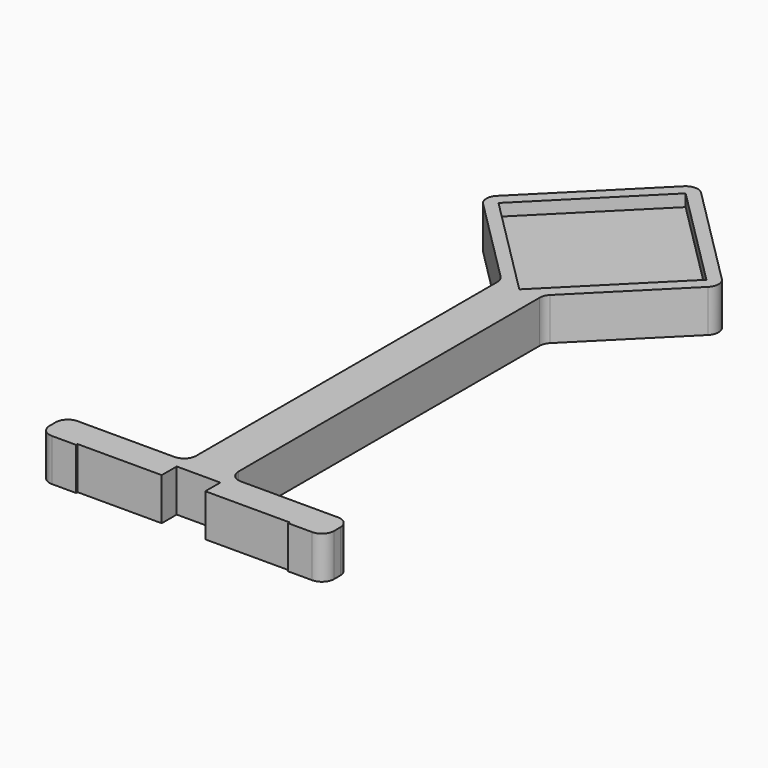
from build123d import *

# Parameters (mm, degrees)
F0_W     = 6
F0_H     = 0.3
F1_DEPTH = 7
F3_DEPTH = 2
F4_R     = 2


# Not quite as in the source:
# - a feature names something its author has since deleted; it is built from what else it names


with BuildPart() as f1:
    # F0 (on Top) → F1 (new body)
    with BuildSketch(Plane.XY):
        Polygon((0, -4), (-3.5, -0.5), (-3.5, -65.5), (-23.5, -65.5), (-23.5, -70.5), (-17.5, -70.5), (-3.6, -70.5), (-3.6, -67.4), (3.6, -67.4), (3.6, -70.5), (17.5, -70.5), (23.5, -70.5), (23.5, -65.5), (3.5, -65.5), (3.5, -0.5), align=None)
        with Locations((-20.5, -70.65)):
            Rectangle(F0_W, F0_H)
        with Locations((20.5, -70.65)):
            Rectangle(F0_W, F0_H)
        Polygon((-20, 16), (-3.5, -0.5), (0, -4), (3.5, -0.5), (20, 16), (0, 36), align=None)
    extrude(amount=F1_DEPTH)

    # F2 (on face) → F3 (cut)
    with BuildSketch(Plane.XY.offset(7)):
        Polygon((0, 33.1715728753), (-17.1715728753, 16), (0, -1.1715728753), (17.1715728753, 16), align=None)
    extrude(amount=-F3_DEPTH, mode=Mode.SUBTRACT)

    # F4
    f4_edges = [f1.edges().sort_by_distance(p)[0] for p in [
        (3.5, -65.5, 3.5),
        (-3.5, -65.5, 3.5),
        (-23.5, -65.5, 3.5),
        (23.5, -65.5, 3.5),
        (-23.5, -70.8, 3.5),
        (23.5, -70.8, 3.5),
        (20, 16, 3.5),
        (0, 36, 3.5),
        (-20, 16, 3.5),
        (3.5, -0.5, 3.5),
        (-3.5, -0.5, 3.5),
    ]]
    fillet(f4_edges, radius=F4_R)


solid = f1.part
